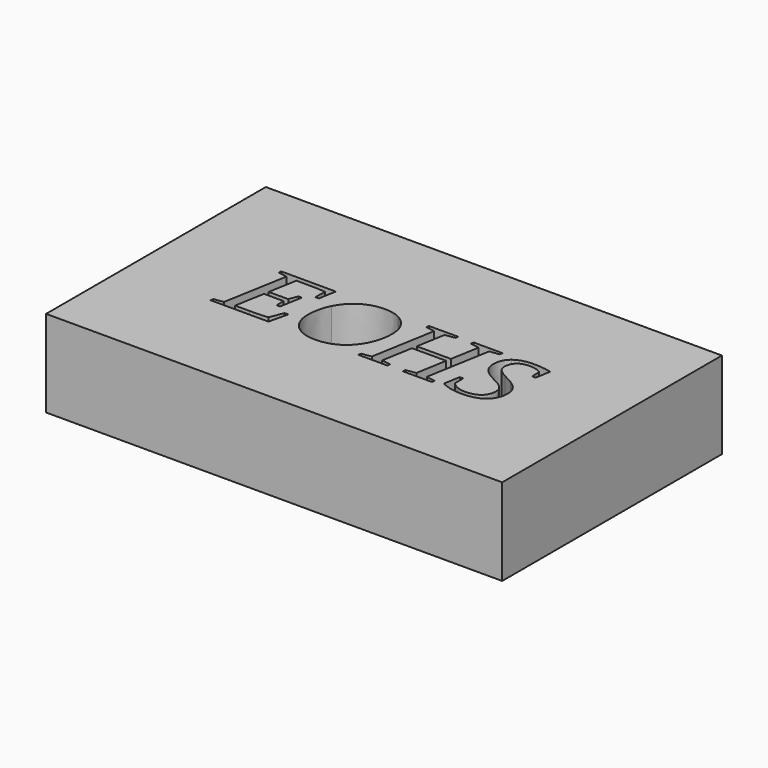
from build123d import *

# Parameters (mm, degrees)
F0_W     = 40.0103181601
F0_H     = 24.0946123376
F1_DEPTH = 7.62


with BuildPart() as f1:
    # F0 (on Top) → F1 (new body)
    with BuildSketch(Plane.XY):
        with Locations((-0.1676287502, 3.8467827253)):
            Rectangle(F0_W, F0_H)
        with BuildLine():
            Line((-11.7563733071, 0.7942912366), (-10.7646722607, 6.4043121633))
            Line((-10.7646722607, 6.4043121633), (-11.5619816778, 6.5273256163))
            Line((-11.5619816778, 6.5273256163), (-11.5133837704, 6.7794272605))
            Line((-11.5133837704, 6.7794272605), (-6.7401580604, 6.7794272605))
            Line((-6.7401580604, 6.7794272605), (-7.0104839199, 5.2561866028))
            Line((-7.0104839199, 5.2561866028), (-7.3233329483, 5.2561866028))
            Line((-7.3233329483, 5.2561866028), (-7.2944779408, 6.2858547642))
            add(Edge.make_bspline(
                [(-7.2944779408, 6.2858547642), (-7.8123493908, 6.3511582022), (-8.8177185985, 6.3511582022)],
                knots=[0, 0, 0, 1, 1, 1], degree=2))
            Line((-8.8177185985, 6.3511582022), (-9.8580175522, 6.3511582022))
            Line((-9.8580175522, 6.3511582022), (-10.2984360873, 3.8650715056))
            Line((-10.2984360873, 3.8650715056), (-8.5808038003, 3.8650715056))
            Line((-8.5808038003, 3.8650715056), (-8.2968097794, 4.6244138076))
            Line((-8.2968097794, 4.6244138076), (-7.9930728586, 4.6244138076))
            Line((-7.9930728586, 4.6244138076), (-8.3393329483, 2.6683480378))
            Line((-8.3393329483, 2.6683480378), (-8.6430698691, 2.6683480378))
            Line((-8.6430698691, 2.6683480378), (-8.6521819767, 3.4383211319))
            Line((-8.6521819767, 3.4383211319), (-10.3698142637, 3.4383211319))
            Line((-10.3698142637, 3.4383211319), (-10.8299756987, 0.8413704593))
            Line((-10.8299756987, 0.8413704593), (-9.5770609005, 0.8413704593))
            add(Edge.make_bspline(
                [(-9.5770609005, 0.8413704593), (-8.3621132174, 0.8413704593), (-7.9596617973, 0.9173046895)],
                knots=[0, 0, 0, 1, 1, 1], degree=2))
            Line((-7.9596617973, 0.9173046895), (-7.4797574625, 2.0942852575))
            Line((-7.4797574625, 2.0942852575), (-7.1669084341, 2.0942852575))
            Line((-7.1669084341, 2.0942852575), (-7.5556916927, 0.4146200856))
            Line((-7.5556916927, 0.4146200856), (-12.6341730081, 0.4146200856))
            Line((-12.6341730081, 0.4146200856), (-12.5870937854, 0.6667217299))
            Line((-12.5870937854, 0.6667217299), (-11.7563733071, 0.7942912366))
        make_face(mode=Mode.SUBTRACT)
        with BuildLine():
            add(Edge.make_bspline(
                [(-1.5644809304, 0.8102374249), (-2.3830519319, 0.3189429556), (-3.437019047, 0.3189429556)],
                knots=[0, 0, 0, 1, 1, 1], degree=2))
            add(Edge.make_bspline(
                [(-3.437019047, 0.3189429556), (-4.2009174027, 0.3189429556), (-4.8106692712, 0.639385407)],
                knots=[0, 0, 0, 1, 1, 1], degree=2))
            add(Edge.make_bspline(
                [(-4.8106692712, 0.639385407), (-5.4204211396, 0.9598278584), (-5.7575691217, 1.5437620886)],
                knots=[0, 0, 0, 1, 1, 1], degree=2))
            add(Edge.make_bspline(
                [(-5.7575691217, 1.5437620886), (-6.0947171038, 2.1276963188), (-6.0947171038, 2.8536275595)],
                knots=[0, 0, 0, 1, 1, 1], degree=2))
            add(Edge.make_bspline(
                [(-6.0947171038, 2.8536275595), (-6.0947171038, 3.9971970662), (-5.6201281651, 4.9251133592)],
                knots=[0, 0, 0, 1, 1, 1], degree=2))
            add(Edge.make_bspline(
                [(-5.6201281651, 4.9251133592), (-5.1455392263, 5.8530296521), (-4.3246901979, 6.3519175445)],
                knots=[0, 0, 0, 1, 1, 1], degree=2))
            add(Edge.make_bspline(
                [(-4.3246901979, 6.3519175445), (-3.5038411695, 6.8508054369), (-2.4498740544, 6.8508054369)],
                knots=[0, 0, 0, 1, 1, 1], degree=2))
            add(Edge.make_bspline(
                [(-2.4498740544, 6.8508054369), (-1.6859756987, 6.8508054369), (-1.0762238302, 6.5303629855)],
                knots=[0, 0, 0, 1, 1, 1], degree=2))
            add(Edge.make_bspline(
                [(-1.0762238302, 6.5303629855), (-0.4664719618, 6.209920534), (-0.1293239797, 5.6282643308)],
                knots=[0, 0, 0, 1, 1, 1], degree=2))
            add(Edge.make_bspline(
                [(-0.1293239797, 5.6282643308), (0.2078240024, 5.0466081275), (0.2078240024, 4.316120833)],
                knots=[0, 0, 0, 1, 1, 1], degree=2))
            add(Edge.make_bspline(
                [(0.2078240024, 4.316120833), (0.2078240024, 3.1907755415), (-0.2690429633, 2.2461537179)],
                knots=[0, 0, 0, 1, 1, 1], degree=2))
            add(Edge.make_bspline(
                [(-0.2690429633, 2.2461537179), (-0.7459099289, 1.3015318943), (-1.5644809304, 0.8102374249)],
                knots=[0, 0, 0, 1, 1, 1], degree=2))
        make_face(mode=Mode.SUBTRACT)
        Polygon((2.8655220592, 0.4146200856), (0.3308374553, 0.4146200856), (0.3688045704, 0.6667217299), (1.2040811025, 0.7942912366), (2.1866700412, 6.4043121633), (1.3984727318, 6.5273256163), (1.4364398469, 6.7794272605), (3.9863112968, 6.7794272605), (3.9483441817, 6.5273256163), (3.0978808036, 6.4043121633), (2.6620183222, 3.9030386207), (5.6568643611, 3.9030386207), (6.0927268424, 6.4043121633), (5.304529533, 6.5273256163), (5.3424966481, 6.7794272605), (7.8908494134, 6.7794272605), (7.8528822983, 6.5273256163), (7.0084936586, 6.4043121633), (6.0259047199, 0.7942912366), (6.8141020293, 0.6667217299), (6.7715788604, 0.4146200856), (4.2277821488, 0.4146200856), (4.2657492639, 0.6667217299), (5.1101379037, 0.7942912366), (5.5809301309, 3.476288247), (2.586084092, 3.476288247), (2.1152918648, 0.7942912366), (2.9034891743, 0.6667217299), align=None, mode=Mode.SUBTRACT)
        with BuildLine():
            Line((7.5688882774, 0.7608801753), (7.8164338678, 2.1747755415))
            Line((7.8164338678, 2.1747755415), (8.1247268424, 2.1747755415))
            Line((8.1247268424, 2.1747755415), (8.1292828962, 1.2696395176))
            add(Edge.make_bspline(
                [(8.1292828962, 1.2696395176), (8.2857074104, 1.0312060348), (8.6631005345, 0.8679474399)],
                knots=[0, 0, 0, 1, 1, 1], degree=2))
            add(Edge.make_bspline(
                [(8.6631005345, 0.8679474399), (9.0404936586, 0.704688845), (9.4626879784, 0.704688845)],
                knots=[0, 0, 0, 1, 1, 1], degree=2))
            add(Edge.make_bspline(
                [(9.4626879784, 0.704688845), (10.2402544956, 0.704688845), (10.6609301309, 1.0722105191)],
                knots=[0, 0, 0, 1, 1, 1], degree=2))
            add(Edge.make_bspline(
                [(10.6609301309, 1.0722105191), (11.0816057662, 1.4397321932), (11.0816057662, 2.0988413113)],
                knots=[0, 0, 0, 1, 1, 1], degree=2))
            add(Edge.make_bspline(
                [(11.0816057662, 2.0988413113), (11.0816057662, 2.3554990094), (10.9677044209, 2.5453345849)],
                knots=[0, 0, 0, 1, 1, 1], degree=2))
            add(Edge.make_bspline(
                [(10.9677044209, 2.5453345849), (10.8538030756, 2.7351701603), (10.6639675001, 2.8870386207)],
                knots=[0, 0, 0, 1, 1, 1], degree=2))
            add(Edge.make_bspline(
                [(10.6639675001, 2.8870386207), (10.4741319246, 3.0389070811), (10.2341797572, 3.1672359302)],
                knots=[0, 0, 0, 1, 1, 1], degree=2))
            add(Edge.make_bspline(
                [(10.2341797572, 3.1672359302), (9.9942275898, 3.2955647792), (9.7428852879, 3.4261716551)],
                knots=[0, 0, 0, 1, 1, 1], degree=2))
            add(Edge.make_bspline(
                [(9.7428852879, 3.4261716551), (9.4915429859, 3.5567785311), (9.2515908185, 3.7063689645)],
                knots=[0, 0, 0, 1, 1, 1], degree=2))
            add(Edge.make_bspline(
                [(9.2515908185, 3.7063689645), (9.0116386511, 3.855959398), (8.8218030756, 4.0526290542)],
                knots=[0, 0, 0, 1, 1, 1], degree=2))
            add(Edge.make_bspline(
                [(8.8218030756, 4.0526290542), (8.6319675001, 4.2492987104), (8.5180661548, 4.5059564085)],
                knots=[0, 0, 0, 1, 1, 1], degree=2))
            add(Edge.make_bspline(
                [(8.5180661548, 4.5059564085), (8.4041648095, 4.7626141065), (8.4041648095, 5.1088741962)],
                knots=[0, 0, 0, 1, 1, 1], degree=2))
            add(Edge.make_bspline(
                [(8.4041648095, 5.1088741962), (8.4041648095, 5.953262836), (8.9782275898, 6.4020341364)],
                knots=[0, 0, 0, 1, 1, 1], degree=2))
            add(Edge.make_bspline(
                [(8.9782275898, 6.4020341364), (9.5522903701, 6.8508054369), (10.6199256466, 6.8508054369)],
                knots=[0, 0, 0, 1, 1, 1], degree=2))
            add(Edge.make_bspline(
                [(10.6199256466, 6.8508054369), (11.4369779635, 6.8508054369), (12.1583531503, 6.670081969)],
                knots=[0, 0, 0, 1, 1, 1], degree=2))
            Line((12.1583531503, 6.670081969), (11.9259944059, 5.3457889944))
            Line((11.9259944059, 5.3457889944), (11.6177014314, 5.3457889944))
            Line((11.6177014314, 5.3457889944), (11.5934024777, 6.1567665729))
            add(Edge.make_bspline(
                [(11.5934024777, 6.1567665729), (11.4415340173, 6.2812987104), (11.1712081578, 6.3663450482)],
                knots=[0, 0, 0, 1, 1, 1], degree=2))
            add(Edge.make_bspline(
                [(11.1712081578, 6.3663450482), (10.9008822983, 6.4513913861), (10.5500661548, 6.4513913861)],
                knots=[0, 0, 0, 1, 1, 1], degree=2))
            add(Edge.make_bspline(
                [(10.5500661548, 6.4513913861), (9.9182933596, 6.4513913861), (9.5765893237, 6.1430984115)],
                knots=[0, 0, 0, 1, 1, 1], degree=2))
            add(Edge.make_bspline(
                [(9.5765893237, 6.1430984115), (9.2348852879, 5.8348054369), (9.2348852879, 5.2789668719)],
                knots=[0, 0, 0, 1, 1, 1], degree=2))
            add(Edge.make_bspline(
                [(9.2348852879, 5.2789668719), (9.2348852879, 4.9797860049), (9.4482604747, 4.7329997568)],
                knots=[0, 0, 0, 1, 1, 1], degree=2))
            add(Edge.make_bspline(
                [(9.4482604747, 4.7329997568), (9.6616356616, 4.4862135086), (10.0838299814, 4.2735976641)],
                knots=[0, 0, 0, 1, 1, 1], degree=2))
            add(Edge.make_bspline(
                [(10.0838299814, 4.2735976641), (10.7292709381, 3.936449682), (11.0140243013, 3.7610416103)],
                knots=[0, 0, 0, 1, 1, 1], degree=2))
            add(Edge.make_bspline(
                [(11.0140243013, 3.7610416103), (11.2987776645, 3.5856335385), (11.4908912669, 3.3859265131)],
                knots=[0, 0, 0, 1, 1, 1], degree=2))
            add(Edge.make_bspline(
                [(11.4908912669, 3.3859265131), (11.6830048693, 3.1862194877), (11.7999435838, 2.9303211319)],
                knots=[0, 0, 0, 1, 1, 1], degree=2))
            add(Edge.make_bspline(
                [(11.7999435838, 2.9303211319), (11.9168822983, 2.6744227762), (11.9168822983, 2.3418308479)],
                knots=[0, 0, 0, 1, 1, 1], degree=2))
            add(Edge.make_bspline(
                [(11.9168822983, 2.3418308479), (11.9168822983, 1.363797963), (11.2782754224, 0.8413704593)],
                knots=[0, 0, 0, 1, 1, 1], degree=2))
            add(Edge.make_bspline(
                [(11.2782754224, 0.8413704593), (10.6396685465, 0.3189429556), (9.433832971, 0.3189429556)],
                knots=[0, 0, 0, 1, 1, 1], degree=2))
            add(Edge.make_bspline(
                [(9.433832971, 0.3189429556), (8.835471237, 0.3189429556), (8.3586042714, 0.4404377239)],
                knots=[0, 0, 0, 1, 1, 1], degree=2))
            add(Edge.make_bspline(
                [(8.3586042714, 0.4404377239), (7.8817373058, 0.5619324922), (7.5688882774, 0.7608801753)],
                knots=[0, 0, 0, 1, 1, 1], degree=2))
        make_face(mode=Mode.SUBTRACT)
    extrude(amount=F1_DEPTH)


solid = f1.part
